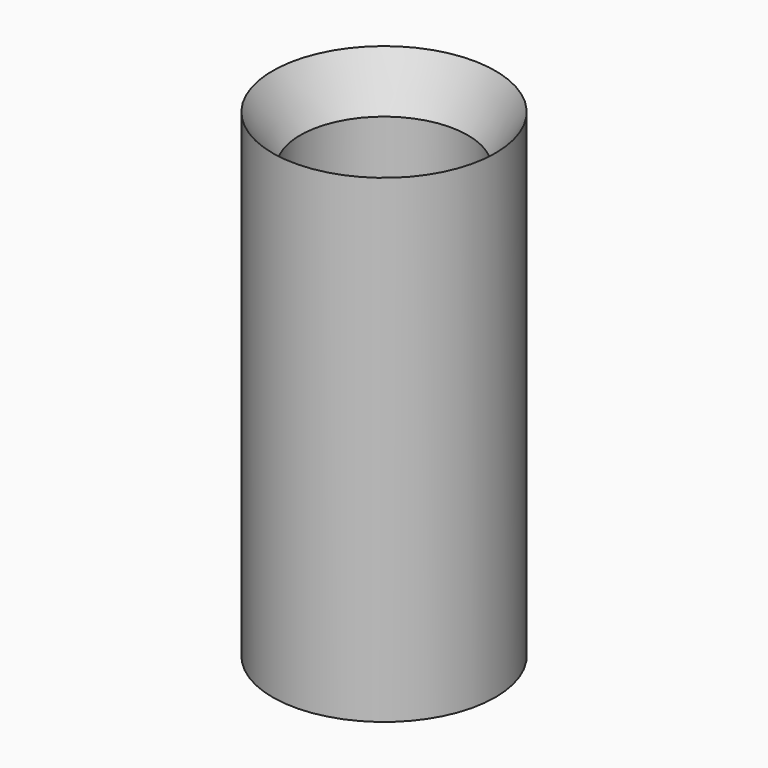
from build123d import *

# Parameters (mm, degrees)
F0_R     = 4.65
F0_R_2   = 3.5
F1_DEPTH = 20


# Not quite as in the source:
# - a fillet or chamfer that OpenCascade refuses, or shapes differently, is made with other operations: its cross-section is extruded or revolved along the edge and cut away or added


with BuildPart() as f1:
    # F0 (on Top) → F1 (new body)
    with BuildSketch(Plane.XY):
        Circle(F0_R)
        Circle(F0_R_2, mode=Mode.SUBTRACT)
    extrude(amount=F1_DEPTH)

    # F2: chamfer of 2 x 1.1547005384 on 1 edges, made by hand

    # F2_s1 → F2_t2 (revolve, cut)
    with BuildSketch(Plane.XZ):
        Polygon((3.5, 18), (4.6547005384, 20), (3.5, 20), align=None)
    revolve(axis=Axis((0, 0, 20), (0, 0, 1)), mode=Mode.SUBTRACT)


solid = f1.part
